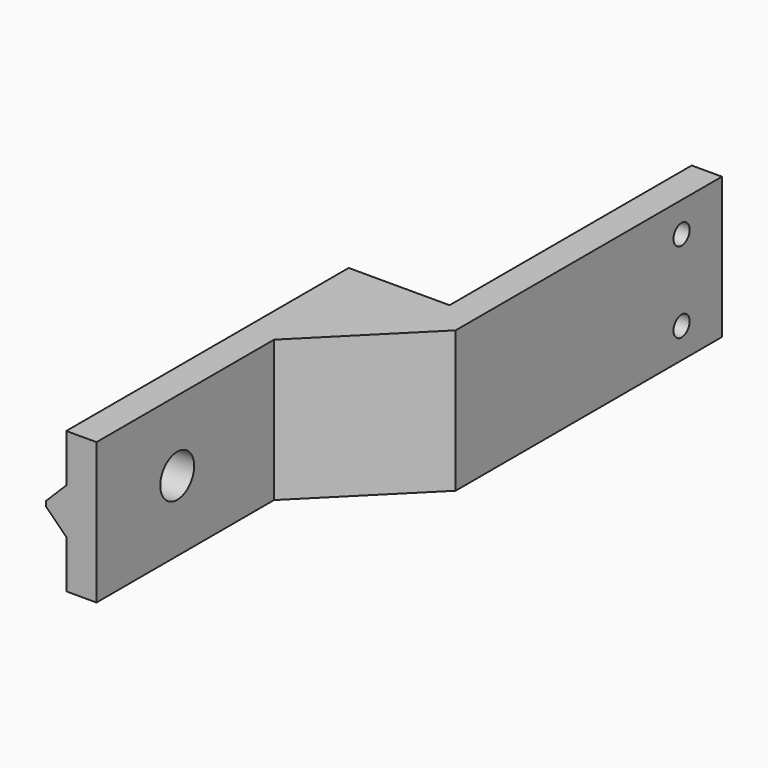
from build123d import *

# Parameters (mm, degrees)
F0_W     = 3
F0_H     = 30
F0_H_2   = 32
F1_DEPTH = 14
F3_D     = 2
F3_DEPTH = 12
F3_TIP   = 0.600860619
F4_W     = 4.5
F4_H     = 4.5
F5_DEPTH = 2
F7_D     = 4.2
F8_SIZE  = 9.99999
F9_SIZE  = 1.99999


# Not quite as in the source:
# - a fillet or chamfer is up to 0.001 mm smaller than in the source, because OpenCascade refuses the exact size


with BuildPart() as f1:
    # F0 (on Top) → F1 (new body)
    with BuildSketch(Plane.XY):
        with Locations((-31.0656790137, 37.4089360237)):
            Rectangle(F0_W, F0_H)
        Polygon((-29.5656790137, 22.4089360237), (-32.5656790137, 22.4089360237), (-42.5656790137, 22.4089360237), (-42.5656790137, 19.4089360237), (-39.5656790137, 19.4089360237), (-29.5656790137, 19.4089360237), align=None)
        with Locations((-41.0656790137, 3.4089360237)):
            Rectangle(F0_W, F0_H_2)
    extrude(amount=F1_DEPTH)

    # F3
    with Locations(Plane.YZ.offset(-29.5656790137)):
        with Locations((47.4089360237, 11), (47.4089360237, 3)):
            Hole(F3_D / 2, depth=F3_DEPTH)
            with Locations((0, 0, -(F3_DEPTH + F3_TIP / 2))):  # 118° drill point
                Cone(0, F3_D / 2, F3_TIP, mode=Mode.SUBTRACT)

    # F4 (on face) → F5 (join)
    with BuildSketch(Plane(origin=(-42.5656790137, 0, 0), x_dir=(0, -1, 0), z_dir=(-1, 0, 0))):
        with Locations((-5.1589360237, 7)):
            Rectangle(F4_W, F4_H)
        with Locations((10.3410639763, 7)):
            Rectangle(F4_W, F4_H)
    extrude(amount=F5_DEPTH)

    # F7 (through all)
    with Locations(Plane.YZ.offset(-39.5656790137)):
        with Locations((-2.5910639763, 7)):
            Hole(F7_D / 2)

    # F8 (size 10 in the source; OpenCascade refuses exactly that, so slightly less here)
    f8_edges = [f1.edges().sort_by_distance(p)[0] for p in [
        (-39.565679, 19.408936, 7),
    ]]
    chamfer(f8_edges, length=F8_SIZE)

    # F9 (size 2 in the source; OpenCascade refuses exactly that, so slightly less here)
    f9_edges = [f1.edges().sort_by_distance(p)[0] for p in [
        (-44.565679, 5.158936, 4.75),
        (-44.565679, -10.341064, 4.75),
        (-44.565679, -10.341064, 9.25),
        (-44.565679, 5.158936, 9.25),
    ]]
    chamfer(f9_edges, length=F9_SIZE)


solid = f1.part
